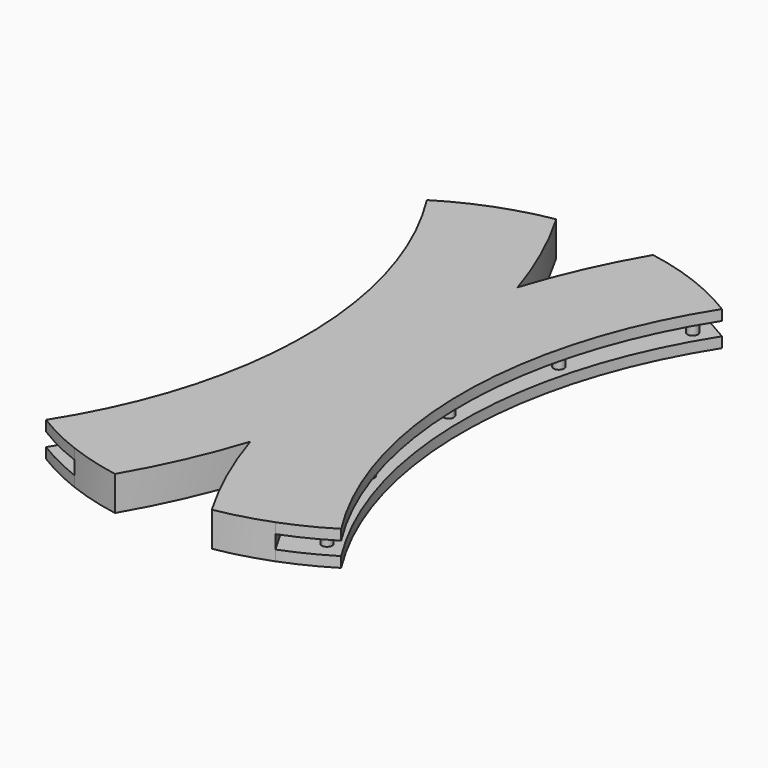
from build123d import *

# Parameters (mm, degrees)
F1_DEPTH = 0.65
F3_DEPTH = 1
F5_R     = 0.5
F6_DEPTH = 3.3


with BuildPart() as f1:
    # F0 (on Top) → F1 (new body, symmetric)
    with BuildSketch(Plane.XY):
        with BuildLine():
            ThreePointArc((59.638121, 25.043336), (57.171718, 25.857852), (54.638121, 26.430095))
            ThreePointArc((54.638121, 26.430095), (52.035138, 21.345304), (50, 16.007811))
            ThreePointArc((50, 16.007811), (51.871235, 8.100926), (52.5, 0))
            ThreePointArc((52.5, 0), (54.319374, 13.020383), (59.638121, 25.043336))
        make_face()
        with BuildLine():
            ThreePointArc((47.5, 0), (48.128765, 8.100926), (50, 16.007811))
            ThreePointArc((50, 16.007811), (47.964862, 21.345304), (45.361879, 26.430095))
            ThreePointArc((45.361879, 26.430095), (42.828282, 25.857852), (40.361879, 25.043336))
            ThreePointArc((40.361879, 25.043336), (45.680626, 13.020383), (47.5, 0))
        make_face()
        with BuildLine():
            ThreePointArc((45.361879, -26.430095), (47.964862, -21.345304), (50, -16.007811))
            ThreePointArc((50, -16.007811), (48.128765, -8.100926), (47.5, 0))
            ThreePointArc((47.5, 0), (45.680626, -13.020383), (40.361879, -25.043336))
            ThreePointArc((40.361879, -25.043336), (42.828282, -25.857852), (45.361879, -26.430095))
        make_face()
        with BuildLine():
            ThreePointArc((50, -16.007811), (52.035138, -21.345304), (54.638121, -26.430095))
            ThreePointArc((54.638121, -26.430095), (57.171718, -25.857852), (59.638121, -25.043336))
            ThreePointArc((59.638121, -25.043336), (54.319374, -13.020383), (52.5, 0))
            ThreePointArc((52.5, 0), (51.871235, -8.100926), (50, -16.007811))
        make_face()
        with BuildLine():
            ThreePointArc((52.5, 0), (51.871235, 8.100926), (50, 16.007811))
            ThreePointArc((50, 16.007811), (48.128765, 8.100926), (47.5, 0))
            ThreePointArc((47.5, 0), (48.128765, -8.100926), (50, -16.007811))
            ThreePointArc((50, -16.007811), (51.871235, -8.100926), (52.5, 0))
        make_face()
    extrude(amount=F1_DEPTH, both=True)

    # F2 (on face) → F3 (join)
    with BuildSketch(Plane(origin=(0, 0, -0.65), x_dir=(1, 0, 0), z_dir=(0, 0, -1))):
        with BuildLine():
            ThreePointArc((35.861879, -22.807359), (38.059426, -24.030912), (40.361879, -25.043336))
            ThreePointArc((40.361879, -25.043336), (45.680626, -13.020383), (47.5, 0))
            ThreePointArc((47.5, 0), (45.680626, 13.020383), (40.361879, 25.043336))
            ThreePointArc((40.361879, 25.043336), (38.059426, 24.030912), (35.861879, 22.807359))
            ThreePointArc((35.861879, 22.807359), (42.5, 0), (35.861879, -22.807359))
        make_face()
        with BuildLine():
            ThreePointArc((47.5, 0), (45.680626, -13.020383), (40.361879, -25.043336))
            ThreePointArc((40.361879, -25.043336), (42.828282, -25.857852), (45.361879, -26.430095))
            ThreePointArc((45.361879, -26.430095), (47.964862, -21.345304), (50, -16.007811))
            ThreePointArc((50, -16.007811), (52.035138, -21.345304), (54.638121, -26.430095))
            ThreePointArc((54.638121, -26.430095), (57.171718, -25.857852), (59.638121, -25.043336))
            ThreePointArc((59.638121, -25.043336), (54.319374, -13.020383), (52.5, 0))
            ThreePointArc((52.5, 0), (54.319374, 13.020383), (59.638121, 25.043336))
            ThreePointArc((59.638121, 25.043336), (57.171718, 25.857852), (54.638121, 26.430095))
            ThreePointArc((54.638121, 26.430095), (52.035138, 21.345304), (50, 16.007811))
            ThreePointArc((50, 16.007811), (47.964862, 21.345304), (45.361879, 26.430095))
            ThreePointArc((45.361879, 26.430095), (42.828282, 25.857852), (40.361879, 25.043336))
            ThreePointArc((40.361879, 25.043336), (45.680626, 13.020383), (47.5, 0))
        make_face()
        with BuildLine():
            ThreePointArc((52.5, 0), (54.319374, -13.020383), (59.638121, -25.043336))
            ThreePointArc((59.638121, -25.043336), (61.940574, -24.030912), (64.138121, -22.807359))
            ThreePointArc((64.138121, -22.807359), (57.5, 0), (64.138121, 22.807359))
            ThreePointArc((64.138121, 22.807359), (61.940574, 24.030912), (59.638121, 25.043336))
            ThreePointArc((59.638121, 25.043336), (54.319374, 13.020383), (52.5, 0))
        make_face()
    extrude(amount=F3_DEPTH)

    # F4: F1 across plane


with BuildPart() as f1_1:
    add(f1.part)
    add(f1.part.mirror(Plane.XY))

    # F5 (on face) → F6 (join, through all)
    with BuildSketch(Plane.XY.offset(1.65)):
        with Locations((37.940756, 21.905106)):
            Circle(F5_R)
        with Locations((42.317414, 11.338917)):
            Circle(F5_R)
        with Locations((43.810211, 0)):
            Circle(F5_R)
        with Locations((42.317414, -11.338917)):
            Circle(F5_R)
        with Locations((37.940756, -21.905106)):
            Circle(F5_R)
        with Locations((62.059244, 21.905106)):
            Circle(F5_R)
        with Locations((57.682586, 11.338917)):
            Circle(F5_R)
        with Locations((56.189789, 0)):
            Circle(F5_R)
        with Locations((57.682586, -11.338917)):
            Circle(F5_R)
        with Locations((62.059244, -21.905106)):
            Circle(F5_R)
    extrude(amount=-F6_DEPTH)


solid = f1_1.part
